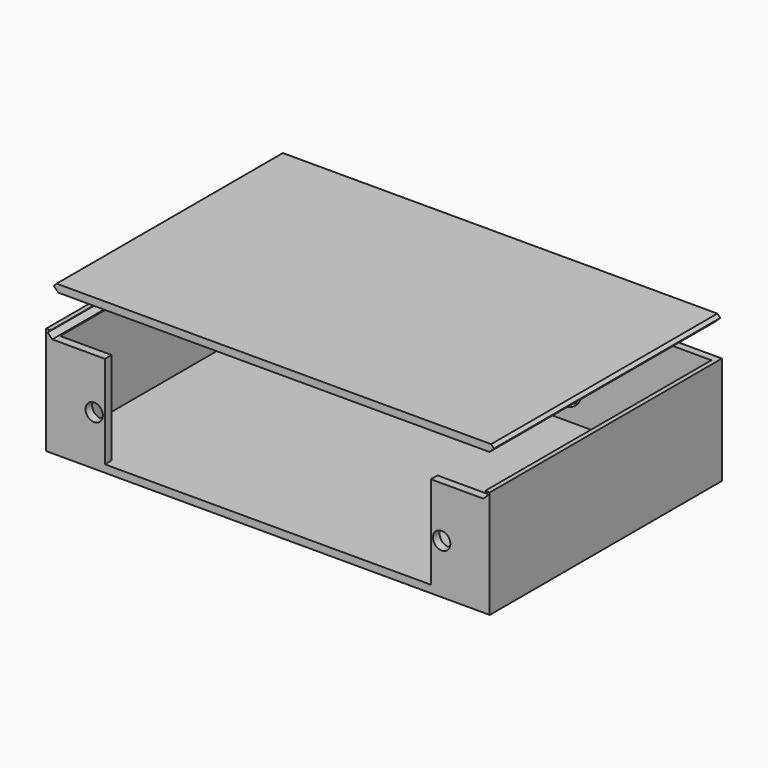
from build123d import *

# Parameters (mm, degrees)
F1_DEPTH = 70
F0_W     = 12.4
F0_H     = 22.4
F0_R     = 2.1
F2_DEPTH = 2
F5_DEPTH = 70
F6_DEPTH = 68.2
F7_R     = 4
F8_DEPTH = 1.8


with BuildPart() as f1:
    # F0 (on Front) → F1 (new body)
    with BuildSketch(Plane.XZ):
        Polygon((-53.5, 0), (-39.3, 0), (-39.3, 1.8), (-51.7, 1.8), (-51.7, 24.2), (-39.3, 24.2), (-39.3, 26), (-53.5, 26), align=None)
        Polygon((0, 24.2), (39.3, 24.2), (39.3, 26), (0, 26), (-39.3, 26), (-39.3, 24.2), align=None)
        Polygon((-39.3, 0), (0, 0), (39.3, 0), (39.3, 1.8), (0, 1.8), (-39.3, 1.8), align=None)
        Polygon((39.3, 1.8), (39.3, 0), (53.5, 0), (53.5, 26), (39.3, 26), (39.3, 24.2), (51.7, 24.2), (51.7, 1.8), align=None)
    extrude(amount=-F1_DEPTH)

    # F0 (on Front) → F2 (join)
    with BuildSketch(Plane.XZ):
        with Locations((45.5, 13)):
            Rectangle(F0_W, F0_H)
        with Locations((41.9, 12)):
            Circle(F0_R, mode=Mode.SUBTRACT)
        with Locations((-45.5, 13)):
            Rectangle(F0_W, F0_H)
        with Locations((-41.9, 12)):
            Circle(F0_R, mode=Mode.SUBTRACT)
    extrude(amount=-F2_DEPTH)

    # F4 (on offset) → F5 (cut)
    with BuildSketch(Plane(origin=(0, 70, 0), x_dir=(-1, 0, 0), z_dir=(0, 1, 0))):
        Polygon((52.4, 26), (0, 26), (-52.4, 26), (-53.1, 25.3), (-52, 24.2), (0, 24.2), (52, 24.2), (53.1, 25.3), align=None)
    extrude(amount=-F5_DEPTH, mode=Mode.SUBTRACT)

    # F7 (on face) → F8 (join)
    with BuildSketch(Plane(origin=(0, 70, 0), x_dir=(-1, 0, 0), z_dir=(0, 1, 0))):
        Polygon((-51.7, 1.8), (0, 1.8), (51.7, 1.8), (51.7, 23.8758921623), (51.7, 24.2), (51.7, 26), (0, 26), (-51.7, 26), (-51.7, 24.2), (-51.7, 23.8758921623), align=None)
        with Locations((-17.0422233641, 8.7407846004)):
            Circle(F7_R, mode=Mode.SUBTRACT)
        with Locations((17.0422233641, 8.7407846004)):
            Circle(F7_R, mode=Mode.SUBTRACT)
        Polygon((51.7, 1.8), (0, 1.8), (-51.7, 1.8), (-51.7, 23.8758921623), (-53.5, 23.8758921623), (-53.5, 0), (53.5, 0), (53.5, 23.8758921623), (51.7, 23.8758921623), align=None)
        Polygon((51.7, 24.2), (51.7, 23.8758921623), (53.5, 23.8758921623), (53.5, 26), (52.4, 26), (53.1, 25.3), (52, 24.2), align=None)
        Polygon((-53.5, 23.8758921623), (-51.7, 23.8758921623), (-51.7, 24.2), (-52, 24.2), (-53.1, 25.3), (-52.4, 26), (-53.5, 26), align=None)
        Polygon((51.7, 26), (51.7, 24.2), (52, 24.2), (53.1, 25.3), (52.4, 26), align=None)
        Polygon((-52, 24.2), (-51.7, 24.2), (-51.7, 26), (-52.4, 26), (-53.1, 25.3), align=None)
    extrude(amount=-F8_DEPTH)


with BuildPart() as f6:
    # F4 (on offset) → F6 (new body)
    with BuildSketch(Plane(origin=(0, 70, 0), x_dir=(-1, 0, 0), z_dir=(0, 1, 0))):
        Polygon((-52, 33.38964656), (0, 33.38964656), (52, 33.38964656), (53.095, 34.48464656), (52.4, 35.17964656), (0, 35.17964656), (-52.4, 35.17964656), (-53.095, 34.48464656), align=None)
    extrude(amount=-F6_DEPTH)


solid = Compound([f1.part, f6.part])
